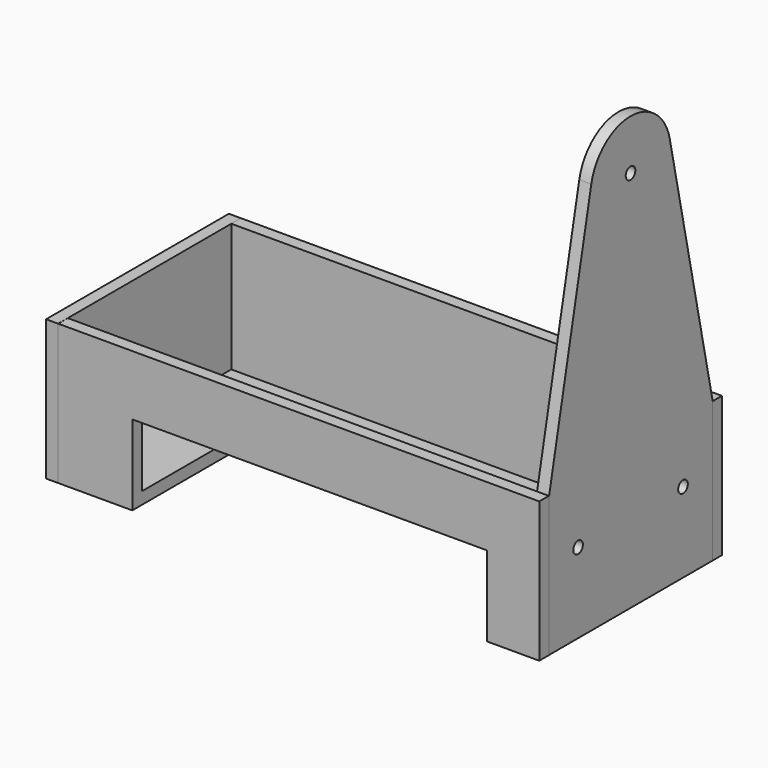
from build123d import *

# Parameters (mm, degrees)
F1_DEPTH  = 3
F3_R      = 1.5
F4_DEPTH  = 3
F7_DEPTH  = 3
F9_W      = 120
F9_H      = 35
F10_DEPTH = 3
F12_W     = 57
F12_H     = 35
F13_DEPTH = 3


with BuildPart() as f1:
    # F0 (on Top) → F1 (new body)
    with BuildSketch(Plane.XY):
        Polygon((58.5, 25.5), (-58.5, 25.5), (-58.5, -25.5), (-40, -25.5), (-40, 10), (48.5, 10), (48.5, -25.5), (58.5, -25.5), align=None)
    extrude(amount=F1_DEPTH)

    # F3 (on offset) → F4 (join)
    with BuildSketch(Plane.YZ.offset(58.5)):
        with BuildLine():
            Line((25.6231492609, 35), (12.2274665574, 98.0959702592))
            ThreePointArc((12.2274665574, 98.0959702592), (-0.0233718405, 107.9999781503), (-12.2370886636, 98.0502276446))
            Line((-12.2370886636, 98.0502276446), (-25.3768507391, 35))
            Line((-25.3768507391, 35), (-25.3768507391, 0))
            Line((-25.3768507391, 0), (25.6231492609, 0))
            Line((25.6231492609, 0), (25.6231492609, 35))
        make_face()
        with Locations((-16.3604691625, 19.9614744633)):
            Circle(F3_R, mode=Mode.SUBTRACT)
        with Locations((16.3604691625, 19.9614744633)):
            Circle(F3_R, mode=Mode.SUBTRACT)
        with Locations((0, 95.5)):
            Circle(F3_R, mode=Mode.SUBTRACT)
    extrude(amount=F4_DEPTH)

    # F6 (on offset) → F7 (join)
    with BuildSketch(Plane.XZ.offset(25.5)):
        Polygon((61.5285639184, 35), (-58.4714360816, 35), (-58.4714360816, 0), (-40, 0), (-40, 20), (48.5, 20), (48.5, 0), (61.5285639184, 0), align=None)
    extrude(amount=F7_DEPTH)

    # F12 (on offset) → F13 (join)
    with BuildSketch(Plane(origin=(-58.5, 0, 0), x_dir=(0, -1, 0), z_dir=(-1, 0, 0))):
        with Locations((0.0093167428, 17.5)):
            Rectangle(F12_W, F12_H)
    extrude(amount=F13_DEPTH)


with BuildPart() as f10:
    # F9 (on offset) → F10 (new body)
    with BuildSketch(Plane(origin=(0, 25.5, 0), x_dir=(-1, 0, 0), z_dir=(0, 1, 0))):
        with Locations((-1.5002019403, 17.5)):
            Rectangle(F9_W, F9_H)
    extrude(amount=F10_DEPTH)


solid = Compound([f1.part, f10.part])
